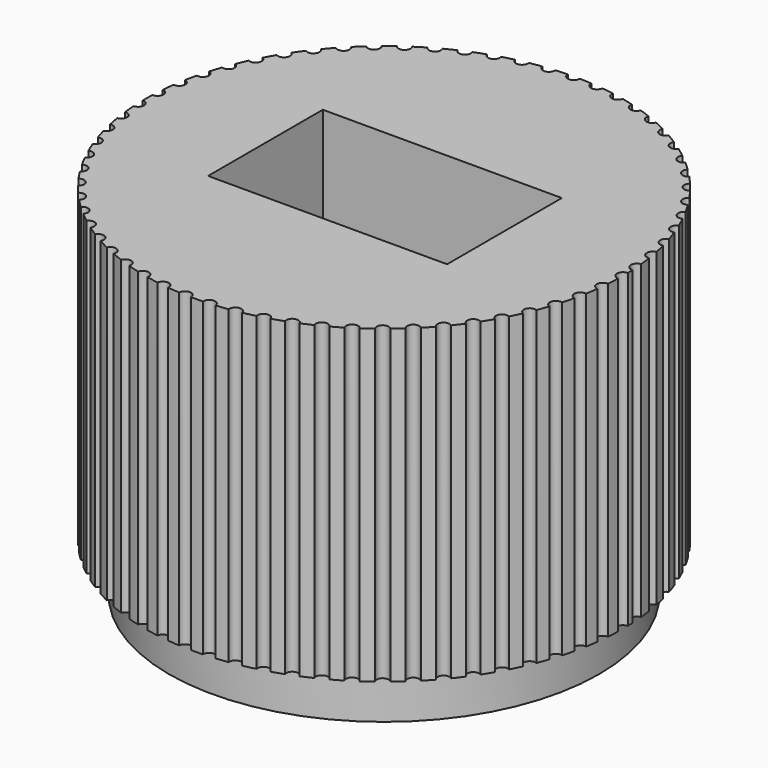
from build123d import *

# Parameters (mm, degrees)
F0_R     = 9
F0_W     = 10
F0_H     = 6
F0_R_2   = 2
F1_DEPTH = 15
F2_START = 2
F2_DEPTH = 13
F3_START = 9
F3_DEPTH = 6


# Not quite as in the source:
# - a feature of the source that left no trace in its solid (it failed there, or was rolled back) is left out


with BuildPart() as f1:
    # F0 (on Top) → F1 (new body)
    with BuildSketch(Plane.XY):
        Circle(F0_R)
        with Locations((0.0031538121, 0.0433453564)):
            Rectangle(F0_W, F0_H, mode=Mode.SUBTRACT)
        with Locations((0.0031538121, 0.0433453564)):
            Rectangle(F0_W, F0_H)
        Circle(F0_R_2, mode=Mode.SUBTRACT)
    extrude(amount=F1_DEPTH)

    # F0 (on Top) → F2 (join)
    with BuildSketch(Plane.XY.offset(F2_START)):
        with BuildLine():
            ThreePointArc((9.996875, -0.249980468), (9.75, 0), (9.996875, 0.249980468))
            ThreePointArc((9.996875, 0.249980468), (9.9927860222, 0.3797729767), (9.9870119794, 0.5095014451))
            ThreePointArc((9.9870119794, 0.5095014451), (9.7218756348, 0.7400230682), (9.9490650435, 1.0080202186))
            ThreePointArc((9.9490650435, 1.0080202186), (9.9207328535, 1.2566064023), (9.8861905026, 1.5044059781))
            ThreePointArc((9.8861905026, 1.5044059781), (9.5993565106, 1.7072945215), (9.7986437778, 1.9966422105))
            ThreePointArc((9.7986437778, 1.9966422105), (9.745625723, 2.241155788), (9.6865071207, 2.4842664513))
            ThreePointArc((9.6865071207, 2.4842664513), (9.3808438212, 2.6574930295), (9.5502360743, 2.9652977802))
            ThreePointArc((9.5502360743, 2.9652977802), (9.4730623354, 3.2032936159), (9.3899586676, 3.43928426))
            ThreePointArc((9.3899586676, 3.43928426), (9.0685226937, 3.5811166072), (9.2063260101, 3.9043003722))
            ThreePointArc((9.2063260101, 3.9043003722), (9.1057683244, 4.1333985075), (8.9995106278, 4.3599092261))
            ThreePointArc((8.9995106278, 4.3599092261), (8.6655163392, 4.4689290188), (8.7703526857, 4.8042599605))
            ThreePointArc((8.7703526857, 4.8042599605), (8.6474166302, 5.0221694141), (8.5190674817, 5.2369351))
            ThreePointArc((8.5190674817, 5.2369351), (8.1758548213, 5.3120521402), (8.2466758346, 5.6561769491))
            ThreePointArc((8.2466758346, 5.6561769491), (8.1025907696, 5.8607186266), (7.9534336609, 6.0615916229))
            ThreePointArc((7.9534336609, 6.0615916229), (7.6044347552, 6.1020547403), (7.640532225, 6.4515321683))
            ThreePointArc((7.640532225, 6.4515321683), (7.4767390014, 6.6406606527), (7.3082655034, 6.8256322295))
            ThreePointArc((7.3082655034, 6.8256322295), (6.9569703416, 6.8310367929), (6.9579832933, 7.1823720657))
            ThreePointArc((6.9579832933, 7.1823720657), (6.7761198432, 7.3541960724), (6.5900146909, 7.5214165138))
            ThreePointArc((6.5900146909, 7.5214165138), (6.2399362245, 7.4917084776), (6.2058545286, 7.8413882425))
            ThreePointArc((6.2058545286, 7.8413882425), (6.0077394865, 7.9941895313), (5.8058637314, 8.141986633))
            ThreePointArc((5.8058637314, 8.141986633), (5.4605027452, 8.0774630776), (5.3916672186, 8.4219905369))
            ThreePointArc((5.3916672186, 8.4219905369), (5.1792817349, 8.5542410949), (4.9636541347, 8.6811368859))
            ThreePointArc((4.9636541347, 8.6811368859), (4.6264642385, 8.5824430467), (4.5235632364, 8.918372926))
            ThreePointArc((4.5235632364, 8.918372926), (4.299031166, 9.0287502476), (4.0718079966, 9.1334757699))
            ThreePointArc((4.0718079966, 9.1334757699), (3.7461610893, 9.0015985854), (3.6102236218, 9.3255715857))
            ThreePointArc((3.6102236218, 9.3255715857), (3.3757902855, 9.4129718978), (3.1392437786, 9.4944798962))
            ThreePointArc((3.1392437786, 9.4944798962), (2.8283963293, 9.3307381382), (2.6607817711, 9.6395145296))
            ThreePointArc((2.6607817711, 9.6395145296), (2.4187915021, 9.703063829), (2.1752871227, 9.7605392235))
            ThreePointArc((2.1752871227, 9.7605392235), (1.882347606, 9.5665703097), (1.6847321026, 9.8570623282))
            ThreePointArc((1.6847321026, 9.8570623282), (1.4376048037, 9.8961251219), (1.1895775957, 9.9289931586))
            ThreePointArc((1.1895775957, 9.9289931586), (0.9174754066, 9.706736778), (0.6918351131, 9.9760395035))
            ThreePointArc((0.6918351131, 9.9760395035), (0.4415537842, 9.9902467565), (0.1909949715, 9.9981758797))
            ThreePointArc((0.1909949715, 9.9981758797), (-0.0575245934, 9.7498303022), (-0.3089572627, 9.995226131))
            ThreePointArc((-0.3089572627, 9.995226131), (-0.5589170849, 9.9843683672), (-0.8085270373, 9.9672606081))
            ThreePointArc((-0.8085270373, 9.9672606081), (-0.8077092229, 9.9556101662), (-0.8074364197, 9.9439342425))
            ThreePointArc((-0.8074364197, 9.9439342425), (-1.0426398182, 9.6943725054), (-1.3056849044, 9.9143929179))
            ThreePointArc((-1.3056849044, 9.9143929179), (-1.5594355808, 9.8776596757), (-1.8121611041, 9.8344329848))
            ThreePointArc((-1.8121611041, 9.8344329848), (-1.8086203944, 9.8103612023), (-1.8074364197, 9.7860592364))
            ThreePointArc((-1.8074364197, 9.7860592364), (-2.0300261522, 9.5375664252), (-2.3014258376, 9.731569201))
            ThreePointArc((-2.3014258376, 9.731569201), (-2.5441659766, 9.6709471865), (-2.7853135236, 9.6042713714))
            ThreePointArc((-2.7853135236, 9.6042713714), (-2.777241426, 9.5683550094), (-2.7745311383, 9.5316426388))
            ThreePointArc((-2.7745311383, 9.5316426388), (-2.9847305146, 9.2848311513), (-3.2618584211, 9.4530566295))
            ThreePointArc((-3.2618584211, 9.4530566295), (-3.4973302405, 9.3684940726), (-3.7306128079, 9.2780670442))
            ThreePointArc((-3.7306128079, 9.2780670442), (-3.7162357574, 9.2309405518), (-3.7113805456, 9.1819096147))
            ThreePointArc((-3.7113805456, 9.1819096147), (-3.9092891294, 8.9373968659), (-4.1896724204, 9.0800134917))
            ThreePointArc((-4.1896724204, 9.0800134917), (-4.415521202, 8.9723560181), (-4.6386059642, 8.8590820466))
            ThreePointArc((-4.6386059642, 8.8590820466), (-4.6162295288, 8.801584344), (-4.6086161474, 8.7403574945))
            ThreePointArc((-4.6086161474, 8.7403574945), (-4.7943642487, 8.4987551487), (-5.0755896956, 8.616170219))
            ThreePointArc((-5.0755896956, 8.616170219), (-5.2895569514, 8.4864944033), (-5.5002130608, 8.3515062286))
            ThreePointArc((-5.5002130608, 8.3515062286), (-5.4682434844, 8.2846713983), (-5.4572655877, 8.2114017994))
            ThreePointArc((-5.4572655877, 8.2114017994), (-5.6310139369, 7.9733142404), (-5.9107510737, 8.0661652441))
            ThreePointArc((-5.9107510737, 8.0661652441), (-6.1106971314, 7.9157678446), (-6.3068180268, 7.7604153482))
            ThreePointArc((-6.3068180268, 7.7604153482), (-6.2637827134, 7.685461146), (-6.2488423722, 7.6003320862))
            ThreePointArc((-6.2488423722, 7.6003320862), (-6.4107817176, 7.3663549055), (-6.6868049411, 7.4354986167))
            ThreePointArc((-6.6868049411, 7.4354986167), (-6.87073034, 7.2658836073), (-7.0503548125, 7.0917203144))
            ThreePointArc((-7.0503548125, 7.0917203144), (-6.9949215356, 7.0100346171), (-6.9754307329, 6.9132590522))
            ThreePointArc((-6.9754307329, 6.9132590522), (-7.125781364, 6.6839775587), (-7.3959907592, 6.7304770032))
            ThreePointArc((-7.3959907592, 6.7304770032), (-7.5620562452, 6.543340534), (-7.7233880501, 6.3521080774))
            ThreePointArc((-7.7233880501, 6.3521080774), (-7.6543826841, 6.2652334073), (-7.6297647863, 6.1570534277))
            ThreePointArc((-7.6297647863, 6.1570534277), (-7.7687759824, 5.9330411839), (-8.0312166696, 5.9581506196))
            ThreePointArc((-8.0312166696, 5.9581506196), (-8.177761588, 5.7553640554), (-8.3191874072, 5.5489747597))
            ThreePointArc((-8.3191874072, 5.5489747597), (-8.2356099925, 5.458591044), (-8.2053011919, 5.3392772689))
            ThreePointArc((-8.2053011919, 5.3392772689), (-8.3332505986, 5.1210946558), (-8.5861304133, 5.1262427299))
            ThreePointArc((-8.5861304133, 5.1262427299), (-8.7116893149, 4.9098339362), (-8.8317948903, 4.6903516943))
            ThreePointArc((-8.8317948903, 4.6903516943), (-8.7328338607, 4.5982574369), (-8.6962845855, 4.4681083374))
            ThreePointArc((-8.6962845855, 4.4681083374), (-8.8134775203, 4.2563011529), (-9.0551828529, 4.2430724128))
            ThreePointArc((-9.0551828529, 4.2430724128), (-9.1585001486, 4.0152054777), (-9.2560844244, 3.784825112))
            ThreePointArc((-9.2560844244, 3.784825112), (-9.1411288438, 3.6929171701), (-9.0978051333, 3.5522583226))
            ThreePointArc((-9.0978051333, 3.5522583226), (-9.2045738215, 3.347356416), (-9.433683464, 3.3174713717))
            ThreePointArc((-9.433683464, 3.3174713717), (-9.5137259809, 3.0804249643), (-9.5878131143, 2.8414502786))
            ThreePointArc((-9.5878131143, 2.8414502786), (-9.4564627897, 2.7517024529), (-9.4058476297, 2.6008857245))
            ThreePointArc((-9.4058476297, 2.6008857245), (-9.5025503738, 2.4034016711), (-9.7178472404, 2.3586956168))
            ThreePointArc((-9.7178472404, 2.3586956168), (-9.7738145533, 2.1148402014), (-9.823663673, 1.8696609424))
            ThreePointArc((-9.823663673, 1.8696609424), (-9.6757370333, 1.7841016007), (-9.6173316498, 1.6235042692))
            ThreePointArc((-9.6173316498, 1.6235042692), (-9.7043519328, 1.4339320881), (-9.9048325444, 1.3763329057))
            ThreePointArc((-9.9048325444, 1.3763329057), (-9.9361649802, 1.1281070364), (-9.961277595, 0.8791749968))
            ThreePointArc((-9.961277595, 0.8791749968), (-9.7968172466, 0.7998639612), (-9.7301423535, 0.6298877711))
            ThreePointArc((-9.7301423535, 0.6298877711), (-9.8078878795, 0.4487016895), (-9.992769523, 0.3802068656))
            ThreePointArc((-9.992769523, 0.3802068656), (-9.9991543081, 0.1300504635), (-9.9992777237, -0.1201873749))
            ThreePointArc((-9.9992777237, -0.1201873749), (-9.8185522598, -0.1911816474), (-9.7431484997, -0.3701122289))
            ThreePointArc((-9.7431484997, -0.3701122289), (-9.8120494448, -0.5424581957), (-9.980773558, -0.6198057626))
            ThreePointArc((-9.980773558, -0.6198057627), (-9.9621436358, -0.869306724), (-9.9372776304, -1.1182635185))
            ThreePointArc((-9.9372776304, -1.1182635185), (-9.7407864983, -1.1788900021), (-9.6562178273, -1.3663265924))
            ThreePointArc((-9.6562178273, -1.3663265924), (-9.7167279895, -1.5294020392), (-9.8689666382, -1.6135357122))
            ThreePointArc((-9.8689666382, -1.6135357122), (-9.8255109765, -1.8599285068), (-9.7759047608, -2.1051570269))
            ThreePointArc((-9.7759047608, -2.1051570269), (-9.5643723957, -2.1534039757), (-9.4702249767, -2.3488776901))
            ThreePointArc((-9.4702249767, -2.3488776901), (-9.522818377, -2.5022746731), (-9.6584700519, -2.5911303047))
            ThreePointArc((-9.6584700519, -2.5911303047), (-9.5906232075, -2.8319510044), (-9.5167728436, -3.0709989651))
            ThreePointArc((-9.5167728436, -3.0709989651), (-9.2911459186, -3.1049181625), (-9.1870298762, -3.3079400108))
            ThreePointArc((-9.1870298762, -3.3079400108), (-9.2322003401, -3.4512747977), (-9.3513887652, -3.5428135941))
            ThreePointArc((-9.3513887652, -3.5428135941), (-9.2598292064, -3.7756539921), (-9.1624731979, -4.0061309136))
            ThreePointArc((-9.1624731979, -4.0061309136), (-8.9239140809, -4.0238608213), (-8.809464477, -4.2339229315))
            ThreePointArc((-8.809464477, -4.2339229315), (-8.8477243987, -4.3668369609), (-8.9507935908, -4.4590687475))
            ThreePointArc((-8.9507935908, -4.4590687475), (-8.8364369133, -4.6816004398), (-8.7165488203, -4.901201553))
            ThreePointArc((-8.7165488203, -4.901201553), (-8.4664266865, -4.9009897348), (-8.341304433, -5.1175666228))
            ThreePointArc((-8.341304433, -5.1175666228), (-8.3731834939, -5.2397274018), (-8.4606904805, -5.3307332135))
            ThreePointArc((-8.4606904805, -5.3307332135), (-8.324680251, -5.5407308831), (-8.1834589545, -5.7472601768))
            ThreePointArc((-8.1834589545, -5.7472601768), (-7.9233386374, -5.7274847631), (-7.7872313447, -5.9500346479))
            ThreePointArc((-7.7872313447, -5.9500346479), (-7.8132751885, -6.0611365834), (-7.8859804654, -6.1490903474))
            ThreePointArc((-7.8859804654, -6.1490903474), (-7.7296767862, -6.3444540175), (-7.5685344992, -6.5358461989))
            ThreePointArc((-7.5685344992, -6.5358461989), (-7.3001631849, -6.4950361678), (-7.152785943, -6.7230023265))
            ThreePointArc((-7.152785943, -6.7230023265), (-7.1735548103, -6.8227674899), (-7.2324106456, -6.9059565777))
            ThreePointArc((-7.2324106456, -6.9059565777), (-7.0573765536, -7.0847326118), (-6.8779246988, -7.2590737589))
            ThreePointArc((-6.8779246988, -7.2590737589), (-6.6032165904, -7.1959278213), (-6.4443126818, -7.4287399819))
            ThreePointArc((-6.4443126818, -7.4287399819), (-6.4603800092, -7.5169188041), (-6.5065167194, -7.5937632423))
            ThreePointArc((-6.5065167194, -7.5937632423), (-6.3145025554, -7.75416388), (-6.1185356515, -7.9097105814))
            ThreePointArc((-6.1185356515, -7.9097105814), (-5.8395547518, -7.8231144696), (-5.6688962938, -8.0601902374))
            ThreePointArc((-5.6688962938, -8.0601902374), (-5.6808472789, -8.1365621335), (-5.7155576259, -8.2056322745))
            ThreePointArc((-5.7155576259, -8.2056322745), (-5.5084835316, -8.3460535094), (-5.2979612476, -8.4812502981))
            ThreePointArc((-5.2979612476, -8.4812502981), (-5.0169024282, -8.3702922758), (-4.8342909428, -8.6110385906))
            ThreePointArc((-4.8342909428, -8.6110385906), (-4.8427210806, -8.6754125114), (-4.8674429563, -8.7354449839))
            ThreePointArc((-4.8674429563, -8.7354449839), (-4.6473796726, -8.8544826037), (-4.4244072313, -8.9679775118))
            ThreePointArc((-4.4244072313, -8.9679775118), (-4.1435757719, -8.8319619385), (-3.9488426825, -9.0757765578))
            ThreePointArc((-3.9488426825, -9.0757765578), (-3.9543562755, -9.1279914677), (-3.970653857, -9.1779032435))
            ThreePointArc((-3.970653857, -9.1779032435), (-3.7398020168, -9.2743668719), (-3.5066091426, -9.3650249504))
            ThreePointArc((-3.5066091426, -9.3650249504), (-3.2283989426, -9.2034837537), (-3.0214059953, -9.4497567595))
            ThreePointArc((-3.0214059953, -9.4497567595), (-3.0246146421, -9.4896820396), (-3.0341582192, -9.5285824707))
            ThreePointArc((-3.0341582192, -9.5285824707), (-2.7948263408, -9.6015074715), (-2.5537449625, -9.6684221394))
            ThreePointArc((-2.5537449626, -9.6684221394), (-2.2806156382, -9.481124069), (-2.0612552481, -9.7292393936))
            ThreePointArc((-2.0612552481, -9.7292393936), (-2.0627763132, -9.7567751682), (-2.0673209992, -9.7839758731))
            ThreePointArc((-2.0673209992, -9.7839758731), (-1.8219024015, -9.8326329963), (-1.5753433329, -9.8751351071))
            ThreePointArc((-1.5753433329, -9.8751351071), (-1.3097964283, -9.6620926669), (-1.0779919485, -9.9114296337))
            ThreePointArc((-1.0779919485, -9.9114296337), (-1.0784470179, -9.9265070203), (-1.0798105692, -9.9415295169))
            ThreePointArc((-1.0798105692, -9.9415295169), (-0.8307594381, -9.9654321911), (-0.5811882698, -9.9830967237))
            ThreePointArc((-0.5811882698, -9.9830967237), (-0.3257428161, -9.7445707009), (-0.0814487294, -9.9945055776))
            ThreePointArc((-0.0814487294, -9.9945055776), (-0.0814620558, -9.9970868591), (-0.0815020335, -9.9996678654))
            ThreePointArc((-0.0815020335, -9.9996678654), (0.1687624158, -9.9985758609), (0.4189211633, -9.9912213998))
            ThreePointArc((0.4189211633, -9.9912213998), (0.6518374888, -9.7281862589), (0.9177635333, -9.9577964479))
            ThreePointArc((0.9177635333, -9.9577964479), (1.1700350551, -9.9313150171), (1.4215537508, -9.8984435612))
            ThreePointArc((1.4215537508, -9.8984435612), (1.6268374888, -9.6133188746), (1.9145059459, -9.8150225157))
            ThreePointArc((1.9145059459, -9.8150225157), (2.1714017029, -9.7614043377), (2.4268020082, -9.7010634475))
            ThreePointArc((2.4268020082, -9.7010634475), (2.6018374888, -9.3964323912), (2.9086326885, -9.5676463084))
            ThreePointArc((2.9086326885, -9.5676463084), (3.1470818219, -9.4918847447), (3.3835609511, -9.4101814696))
            ThreePointArc((3.3835609511, -9.4101814696), (3.5272962514, -9.0895919135), (3.8496574517, -9.2293086147))
            ThreePointArc((3.8496574517, -9.2293086147), (4.0793476591, -9.1301107702), (4.3064842845, -9.0251976769))
            ThreePointArc((4.3064842845, -9.0251976769), (4.4174820515, -8.6918555168), (4.7521856404, -8.7986778347))
            ThreePointArc((4.7521856404, -8.7986778347), (4.9708200198, -8.677035688), (5.1863427751, -8.5499619075))
            ThreePointArc((5.1863427751, -8.5499619075), (5.2634930311, -8.2072005648), (5.6071919727, -8.2800602765))
            ThreePointArc((5.6071919727, -8.2800602765), (5.8125841803, -8.1371902489), (6.0143378379, -7.9892265189))
            ThreePointArc((6.0143378379, -7.9892265189), (6.0568690804, -7.6404736073), (6.4061263852, -7.6786421154))
            ThreePointArc((6.4061263852, -7.6786421154), (6.596222499, -7.5159729073), (6.7821895224, -7.3485988652))
            ThreePointArc((6.7821895224, -7.3485988652), (6.7896764388, -6.9973419136), (7.1409995339, -7.0004375332))
            ThreePointArc((7.1409995339, -7.0004375332), (7.3138985927, -6.8195958367), (7.4822193116, -6.6344852229))
            ThreePointArc((7.4822193116, -6.6344852229), (7.4545870329, -6.2842368008), (7.8044626873, -6.2522285757))
            ThreePointArc((7.8044626873, -6.2522285757), (7.9584357005, -6.0550228076), (8.1074269077, -5.8540267283))
            ThreePointArc((8.1074269077, -5.8540267283), (8.0449517567, -5.50828932), (8.3898812138, -5.4414973324))
            ThreePointArc((8.3898812138, -5.4414973324), (8.5233884513, -5.2298995505), (8.6515602348, -5.0150279664))
            ThreePointArc((8.6515602348, -5.0150279664), (8.5548669628, -4.677258946), (8.8914009281, -4.5763511158))
            ThreePointArc((8.8914009281, -4.5763511158), (9.0031073175, -4.352477298), (9.1091779595, -4.1258789249))
            ThreePointArc((9.1091779595, -4.1258789249), (8.9792334994, -3.7994559826), (9.3040066332, -3.665441388))
            ThreePointArc((9.3040066332, -3.665441388), (9.3927951106, -3.4315302724), (9.4757039045, -3.1954710941))
            ThreePointArc((9.4757039045, -3.1954710941), (9.313807701, -2.8836584593), (9.623572272, -2.7178772464))
            ThreePointArc((9.623572272, -2.7178772464), (9.6885549526, -2.4762679441), (9.7474728106, -2.2331085524))
            ThreePointArc((9.7474728106, -2.2331085524), (9.5552438255, -1.9390243514), (9.846902188, -1.7431343323))
            ThreePointArc((9.846902188, -1.7431343323), (9.887429245, -1.4962429363), (9.9217669885, -1.2484149252))
            ThreePointArc((9.9217669885, -1.2484149252), (9.7011275118, -0.975), (9.9717630821, -0.7509600748))
            ThreePointArc((9.9717630821, -0.7509600748), (9.9874607311, -0.5006277506), (9.996875, -0.249980468))
        make_face()
        Circle(F0_R, mode=Mode.SUBTRACT)
    extrude(amount=F2_DEPTH)

    # F0 (on Top) → F3 (cut)
    with BuildSketch(Plane.XY.offset(F3_START)):
        with Locations((0.0031538121, 0.0433453564)):
            Rectangle(F0_W, F0_H)
        Circle(F0_R_2, mode=Mode.SUBTRACT)
    extrude(amount=F3_DEPTH, mode=Mode.SUBTRACT)


solid = f1.part
